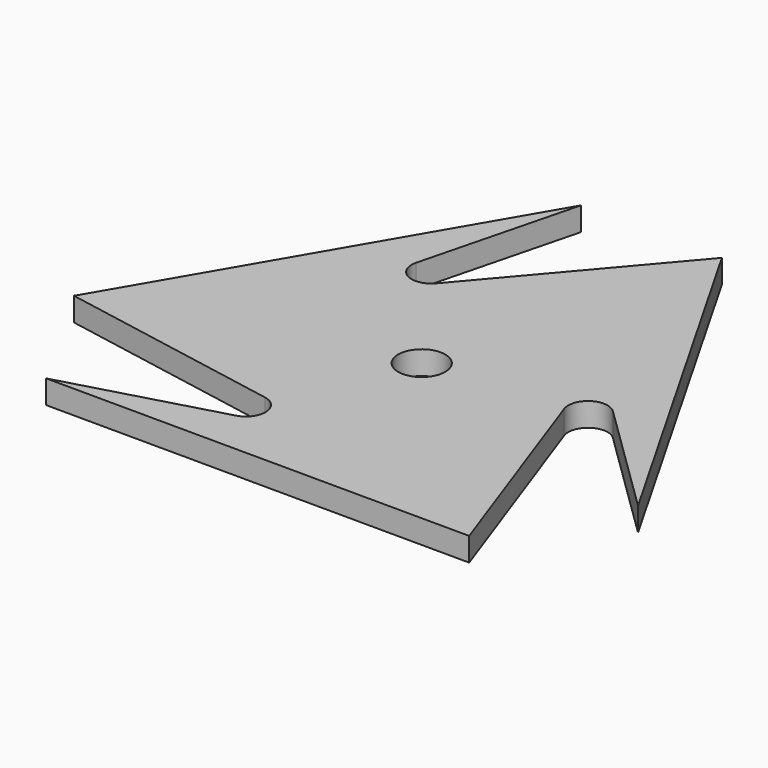
from build123d import *

# Parameters (mm, degrees)
F0_R     = 3
F1_DEPTH = 3
F2_DEPTH = 3
F3_R     = 2.5
F4_R     = 2.5
F5_R     = 2.5


# Not quite as in the source:
# - a feature names something its author has since deleted; it is built from what else it names


with BuildPart() as f1:
    # F0 (on Top) → F1 (new body)
    with BuildSketch(Plane.XY):
        Polygon((73.486745642, 26.9546627321), (46.6403742633, 73.8689917145), (20.8729718881, 43.5791923222), (28.6391571445, 73.9381045595), (1.4333421336, 27.2313004548), (40.5487790704, 20.0609751046), (10.3740972135, 11.6072327084), (64.4262836031, 11.3997078307), (51.0782490415, 48.8598325732), align=None)
        with Locations((37.5, 37.5)):
            Circle(F0_R, mode=Mode.SUBTRACT)
    extrude(amount=F1_DEPTH)

    # F0 (on Top) → F2 (join)
    with BuildSketch(Plane.XY):
        Polygon((73.486745642, 26.9546627321), (46.6403742633, 73.8689917145), (20.8729718881, 43.5791923222), (28.6391571445, 73.9381045595), (1.4333421336, 27.2313004548), (40.5487790704, 20.0609751046), (10.3740972135, 11.6072327084), (64.4262836031, 11.3997078307), (51.0782490415, 48.8598325732), align=None)
        with Locations((37.5, 37.5)):
            Circle(F0_R, mode=Mode.SUBTRACT)
    extrude(amount=F2_DEPTH)

    # F3
    f3_edges = [f1.edges().sort_by_distance(p)[0] for p in [
        (51.078249, 48.859833, 1.5),
    ]]
    fillet(f3_edges, radius=F3_R)

    # F4
    f4_edges = [f1.edges().sort_by_distance(p)[0] for p in [
        (20.872972, 43.579192, 1.5),
    ]]
    fillet(f4_edges, radius=F4_R)

    # F5
    f5_edges = [f1.edges().sort_by_distance(p)[0] for p in [
        (40.548779, 20.060975, 1.5),
    ]]
    fillet(f5_edges, radius=F5_R)


solid = f1.part
